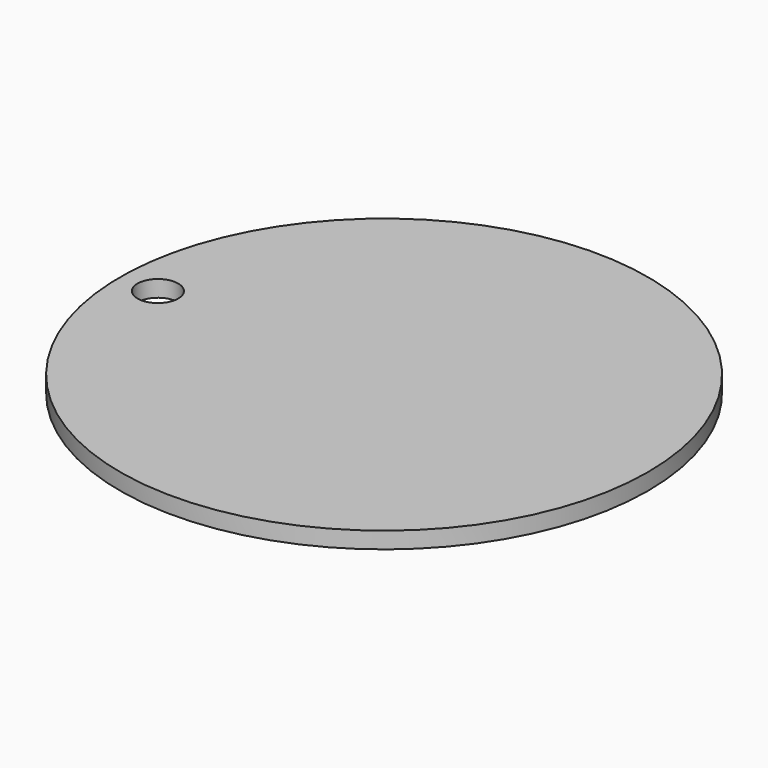
from build123d import *

# Parameters (mm, degrees)
F0_R     = 50.8
F1_DEPTH = 3.175
F2_R     = 3.9184607148
F3_DEPTH = 25.4


# Not quite as in the source:
# - a length typed as a fraction of an inch, garbled in the dataset ("3 / 203.2 mm" for 3/8 in), is restored


with BuildPart() as f1:
    # F0 (on Top) → F1 (new body)
    with BuildSketch(Plane.XY):
        Circle(F0_R)
    extrude(amount=F1_DEPTH)

    # F2 (on face) → F3 (cut)
    with BuildSketch(Plane.XY.offset(3.175)):
        with Locations((-43.5310043395, 0)):
            Circle(F2_R)
    extrude(amount=-F3_DEPTH, mode=Mode.SUBTRACT)


solid = f1.part
